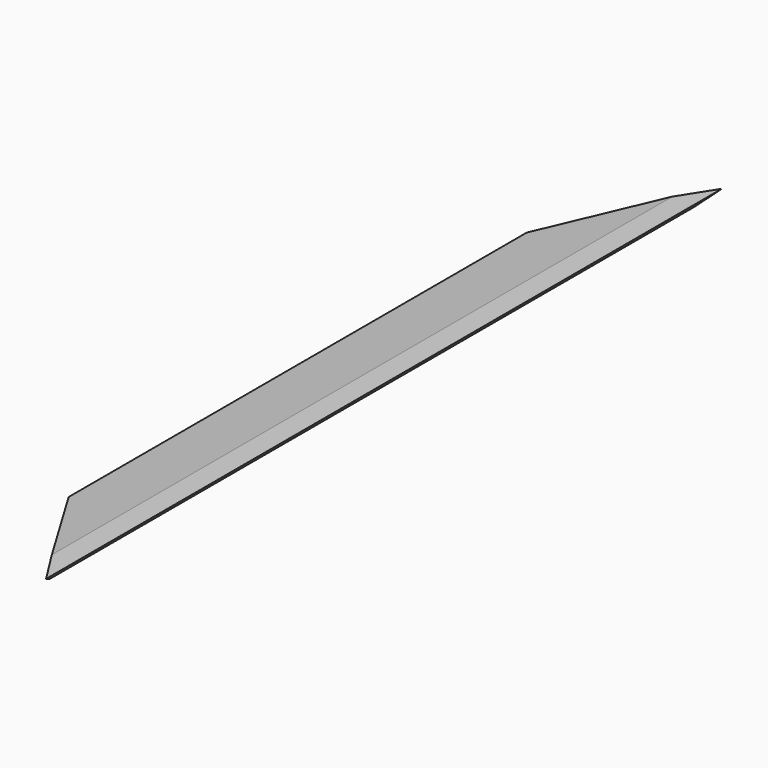
from build123d import *

# Parameters (mm, degrees)
F1_DEPTH = 6.35
F2_SIZE  = 6.34999
F3_SIZE2 = 6.0462521685
F3_SIZE  = 34.29


# Not quite as in the source:
# - a fillet or chamfer is up to 0.001 mm smaller than in the source, because OpenCascade refuses the exact size


with BuildPart() as f1:
    # F0 (on Top) → F1 (new body)
    with BuildSketch(Plane.XY):
        Polygon((75, -225), (75, 225), (29.020415619, 152.489066124), (29.020415619, -152.489066124), align=None)
    extrude(amount=F1_DEPTH)

    # F2 (size 6.35 in the source; OpenCascade refuses exactly that, so slightly less here)
    f2_edges = [f1.edges().sort_by_distance(p)[0] for p in [
        (75, 0, 0),
    ]]
    chamfer(f2_edges, length=F2_SIZE)

    # F3
    f3_edges = [f1.edges().sort_by_distance(p)[0] for p in [
        (29.020416, 0, 6.35),
    ]]
    f3_side = f1.faces().sort_by_distance((53.482225, 0, 6.35))[0]
    chamfer(f3_edges, length=F3_SIZE, length2=F3_SIZE2, reference=f3_side)


solid = f1.part
